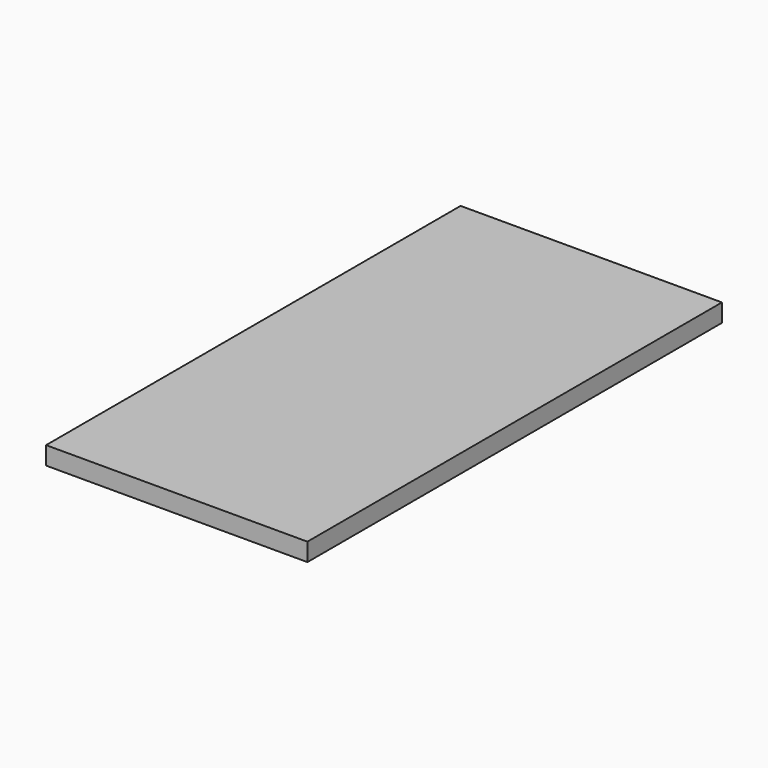
from build123d import *

# Parameters (mm, degrees)
F0_W     = 3683
F0_H     = 7302.5
F1_DEPTH = 254
F2_DEPTH = 101.6
F3_W     = 558.8
F3_H     = 901.7
F3_W_2   = 231.775
F3_H_2   = 1168.4
F3_W_3   = 511.175
F3_H_3   = 546.1
F3_W_4   = 225.425
F4_DEPTH = 50.8


# Not quite as in the source:
# - a feature names something its author has since deleted; it is built from what else it names


with BuildPart() as f1:
    # F0 (on Top) → F1 (new body)
    with BuildSketch(Plane.XY):
        with Locations((-1555.75, 3365.5)):
            Rectangle(F0_W, F0_H)
        Polygon((0, 5156.2), (0, 0), (-2343.15, 0), (-2343.15, 2794), (-3232.15, 2794), (-3232.15, 3810), (-2946.4, 3810), (-2946.4, 6731), (0, 6731), (0, 5899.15), (-34.925, 5899.15), (-34.925, 5156.2), align=None, mode=Mode.SUBTRACT)
    extrude(amount=-F1_DEPTH)

    # F0 (on Top) → F2 (join)
    with BuildSketch(Plane.XY):
        with Locations((-1555.75, 3365.5)):
            Rectangle(F0_W, F0_H)
        Polygon((0, 5156.2), (0, 0), (-2343.15, 0), (-2343.15, 2794), (-3232.15, 2794), (-3232.15, 3810), (-2946.4, 3810), (-2946.4, 6731), (0, 6731), (0, 5899.15), (-34.925, 5899.15), (-34.925, 5156.2), align=None, mode=Mode.SUBTRACT)
        Polygon((-2343.15, 0), (0, 0), (0, 5156.2), (-34.925, 5156.2), (-34.925, 5899.15), (0, 5899.15), (0, 6731), (-2946.4, 6731), (-2946.4, 3810), (-3232.15, 3810), (-3232.15, 2794), (-2343.15, 2794), align=None)
    extrude(amount=-F2_DEPTH)

    # F3 (on face) → F4 (cut)
    with BuildSketch(Plane(origin=(0, 0, -101.6), x_dir=(1, 0, 0), z_dir=(0, 0, -1))):
        with Locations((-1781.175, -450.85)):
            Rectangle(F3_W, F3_H)
        with Locations((-1171.575, -450.85)):
            Rectangle(F3_W, F3_H)
        with Locations((-561.975, -450.85)):
            Rectangle(F3_W, F3_H)
        with Locations((-115.8875, -450.85)):
            Rectangle(F3_W_2, F3_H)
        with Locations((-115.8875, -1536.7)):
            Rectangle(F3_W_2, F3_H_2)
        Polygon((-2111.375, -2171.7), (-2343.15, -2171.7), (-2343.15, -2794), (-2670.175, -2794), (-2670.175, -3340.1), (-2111.375, -3340.1), align=None)
        with Locations((-2976.5625, -3067.05)):
            Rectangle(F3_W_3, F3_H_3)
        with Locations((-115.8875, -3975.1)):
            Rectangle(F3_W_2, F3_H_2)
        with Locations((-2833.6875, -5194.3)):
            Rectangle(F3_W_4, F3_H_2)
        with Locations((-2227.2625, -450.85)):
            Rectangle(F3_W_2, F3_H)
        with Locations((-2227.2625, -1536.7)):
            Rectangle(F3_W_2, F3_H_2)
        with Locations((-1781.175, -1536.7)):
            Rectangle(F3_W, F3_H_2)
        with Locations((-1171.575, -1536.7)):
            Rectangle(F3_W, F3_H_2)
        with Locations((-561.975, -1536.7)):
            Rectangle(F3_W, F3_H_2)
        with Locations((-1781.175, -2755.9)):
            Rectangle(F3_W, F3_H_2)
        with Locations((-1171.575, -2755.9)):
            Rectangle(F3_W, F3_H_2)
        with Locations((-561.975, -2755.9)):
            Rectangle(F3_W, F3_H_2)
        with Locations((-115.8875, -2755.9)):
            Rectangle(F3_W_2, F3_H_2)
        Polygon((-2720.975, -3390.9), (-3232.15, -3390.9), (-3232.15, -3810), (-2946.4, -3810), (-2946.4, -4559.3), (-2720.975, -4559.3), align=None)
        with Locations((-2390.775, -3975.1)):
            Rectangle(F3_W, F3_H_2)
        with Locations((-1781.175, -3975.1)):
            Rectangle(F3_W, F3_H_2)
        with Locations((-1171.575, -3975.1)):
            Rectangle(F3_W, F3_H_2)
        with Locations((-561.975, -3975.1)):
            Rectangle(F3_W, F3_H_2)
        with Locations((-2390.775, -5194.3)):
            Rectangle(F3_W, F3_H_2)
        with Locations((-1781.175, -5194.3)):
            Rectangle(F3_W, F3_H_2)
        with Locations((-1171.575, -5194.3)):
            Rectangle(F3_W, F3_H_2)
        with Locations((-561.975, -5194.3)):
            Rectangle(F3_W, F3_H_2)
        Polygon((0, -5156.2), (0, -4610.1), (-231.775, -4610.1), (-231.775, -5778.5), (-34.925, -5778.5), (-34.925, -5156.2), align=None)
        with Locations((-2833.6875, -6280.15)):
            Rectangle(F3_W_4, F3_H)
        with Locations((-2390.775, -6280.15)):
            Rectangle(F3_W, F3_H)
        with Locations((-1781.175, -6280.15)):
            Rectangle(F3_W, F3_H)
        with Locations((-1171.575, -6280.15)):
            Rectangle(F3_W, F3_H)
        with Locations((-561.975, -6280.15)):
            Rectangle(F3_W, F3_H)
        Polygon((-34.925, -5899.15), (-34.925, -5829.3), (-231.775, -5829.3), (-231.775, -6731), (0, -6731), (0, -5899.15), align=None)
    extrude(amount=-F4_DEPTH, mode=Mode.SUBTRACT)


solid = f1.part
